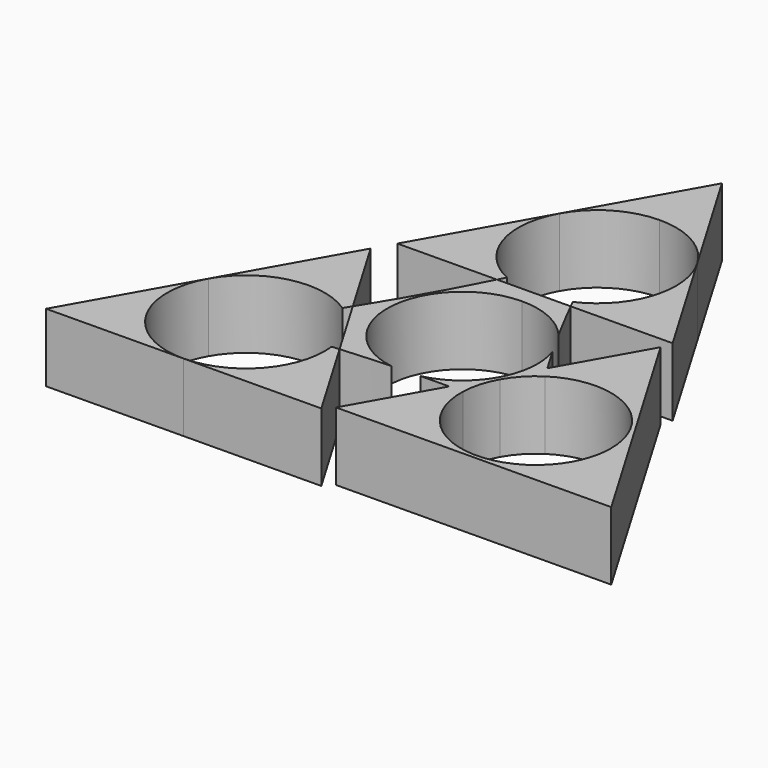
from build123d import *

# Parameters (mm, degrees)
F1_DEPTH = 10


with BuildPart() as f1:
    # F0 (on Top) → F1 (new body)
    with BuildSketch(Plane.XY):
        with BuildLine():
            ThreePointArc((-9.4724629741, -5.5921771434), (-9.5791989557, 5.4073050003), (-0.1067359816, 10.9994821437))
            Line((-0.1067359816, 10.9994821437), (-0.1305380532, 13.4523612782))
            Line((-0.1305380315, 13.4523612785), (-5.6676372798, 13.3986307741))
            ThreePointArc((-5.6676372798, 13.3986307741), (-9.8619346797, 5.5669048062), (-14.3998991761, -2.070826568))
            Line((-14.3998991761, -2.070826568), (-11.5848176191, -6.8392298452))
            Line((-11.5848175812, -6.8392299094), (-9.4724629741, -5.5921771434))
        make_face()
        with BuildLine():
            Line((-0.1305380532, 13.4523612782), (-0.1067359816, 10.9994821437))
            ThreePointArc((-0.1067359816, 10.9994821437), (4.5895542781, 9.9967990641), (8.4111545556, 7.0888982954))
            ThreePointArc((8.4111545556, 7.0888982954), (6.7054289822, 10.2806322034), (5.0577336181, 13.5027068547))
            Line((5.0577336181, 13.5027068547), (-0.1305380315, 13.4523612785))
        make_face()
        with BuildLine():
            ThreePointArc((-1.7230864536, -10.8642060489), (-6.1873786002, -9.0948527233), (-9.4724629741, -5.5921771434))
            Line((-9.4724629741, -5.5921771434), (-11.5848175812, -6.8392299094))
            Line((-11.5848176191, -6.8392298452), (-8.9470811973, -11.3072321903))
            ThreePointArc((-8.9470811973, -11.3072321903), (-5.3370880091, -11.0530388546), (-1.7230864536, -10.8642060489))
        make_face()
    extrude(amount=F1_DEPTH)


with BuildPart() as f1b:
    # F0 (on Top) → F1, piece 2 (new body)
    with BuildSketch(Plane.XY):
        with BuildLine():
            Line((12.5545481824, -0.1363868252), (9.5791989174, -5.4073050681))
            Line((9.5791989557, -5.4073050003), (10.0555510831, -5.6761981773))
            ThreePointArc((10.0555510831, -5.6761981773), (11.606819874, -3.563374371), (13.6139198008, -1.8775484067))
            ThreePointArc((13.6139198008, -1.8775484067), (13.0820160477, -1.0083170753), (12.5545481824, -0.1363868252))
        make_face()
        with BuildLine():
            Line((6.6038497291, -10.6782231755), (9.5791989174, -5.4073050681))
            ThreePointArc((9.5791989174, -5.4073050681), (6.5679269383, -8.8239637201), (2.4308083201, -10.7280553182))
            ThreePointArc((2.4308083201, -10.7280553182), (4.517199042, -10.692254253), (6.6038497291, -10.6782231755))
        make_face()
        with BuildLine():
            Line((10.0555510831, -5.6761981773), (9.5791989557, -5.4073050003))
            Line((9.5791989174, -5.4073050681), (6.6038497291, -10.6782231755))
            ThreePointArc((6.6038497291, -10.6782231755), (7.6229098775, -10.6792833185), (8.6419513958, -10.6855358516))
            ThreePointArc((8.6419513958, -10.6855358516), (9.0481954867, -8.0960523053), (10.0555510831, -5.6761981773))
        make_face()
        with BuildLine():
            ThreePointArc((11, 0), (10.6388718408, -2.7954258985), (9.5791989174, -5.4073050681))
            Line((9.5791989174, -5.4073050681), (12.5545481824, -0.1363868252))
            ThreePointArc((12.5545481824, -0.1363868252), (11.4883643789, 1.6573690273), (10.4409534845, 3.4621511137))
            ThreePointArc((10.4409534845, 3.4621511137), (10.8593390298, 1.7534981708), (11, 0))
        make_face()
        with BuildLine():
            ThreePointArc((8.6419513958, -10.6855358516), (7.6229098775, -10.6792833185), (6.6038497291, -10.6782231755))
            Line((6.6038497291, -10.6782231755), (-0.2522646812, -22.8240303744))
            Line((-0.2522646812, -22.8240303744), (39.7458522051, -22.4358995322))
            Line((39.7458522051, -22.4358995322), (19.4106625927, 12.0094203738))
            Line((19.4106625927, 12.0094203738), (12.5545481824, -0.1363868252))
            ThreePointArc((12.5545481824, -0.1363868252), (13.0820160477, -1.0083170753), (13.6139198008, -1.8775484067))
            ThreePointArc((13.6139198008, -1.8775484067), (24.8678594101, -1.4080411055), (30.6347500389, -11.0835031776))
            ThreePointArc((30.6347500389, -11.0835031776), (30.2736218896, -13.8789290385), (29.2139489946, -16.4908081779))
            ThreePointArc((29.2139489946, -16.4908081779), (16.6472991665, -21.6700577298), (8.6419513958, -10.6855358516))
        make_face()
    extrude(amount=F1_DEPTH)


with BuildPart() as f1c:
    # F0 (on Top) → F1, piece 3 (new body)
    with BuildSketch(Plane.XY):
        with BuildLine():
            ThreePointArc((-5.6676372798, 13.3986307741), (-5.3835781261, 13.9607653638), (-5.1012906228, 14.5237917089))
            ThreePointArc((-5.1012906228, 14.5237917089), (-11.2345943606, 21.4620176196), (-10.2981329222, 30.6750211202))
            Line((-10.2981329222, 30.6750211202), (-20.1295964964, 13.2582958572))
            Line((-20.1295964964, 13.2582958572), (-5.6676372798, 13.3986307741))
        make_face()
    extrude(amount=F1_DEPTH)


with BuildPart() as f1d:
    # F0 (on Top) → F1, piece 4 (new body)
    with BuildSketch(Plane.XY):
        with BuildLine():
            ThreePointArc((11.3044236075, 24.9988230539), (9.473956651, 18.7600560024), (4.5628983325, 14.4992661939))
            ThreePointArc((4.5628983325, 14.4992661939), (4.8096229597, 14.0006424117), (5.0577336181, 13.5027068547))
            Line((5.0577336181, 13.5027068547), (19.8685203899, 13.6464266993))
            Line((19.8685203899, 13.6464266993), (9.7009257177, 30.8690864252))
            ThreePointArc((9.7009257177, 30.8690864252), (10.8963380075, 28.0414862595), (11.3044236075, 24.9988230539))
        make_face()
    extrude(amount=F1_DEPTH)


with BuildPart() as f1e:
    # F0 (on Top) → F1, piece 5 (new body)
    with BuildSketch(Plane.XY):
        with BuildLine():
            ThreePointArc((-8.9470811973, -11.3072321903), (-9.501595119, -11.3520989755), (-10.0559820928, -11.3985080385))
            ThreePointArc((-10.0559820928, -11.3985080385), (-10.0000003021, -12.0529385986), (-9.9813195575, -12.7094935078))
            ThreePointArc((-9.9813195575, -12.7094935078), (-13.3238411908, -20.8347491789), (-21.4162808358, -24.2559552797))
            Line((-21.4162808358, -24.2559552797), (-1.417222775, -24.0618898624))
            Line((-1.417222775, -24.0618898624), (-8.9470811973, -11.3072321903))
        make_face()
    extrude(amount=F1_DEPTH)


with BuildPart() as f1f:
    # F0 (on Top) → F1, piece 6 (new body)
    with BuildSketch(Plane.XY):
        with BuildLine():
            ThreePointArc((-31.5838762413, -7.0332957148), (-24.1799561682, -1.471069011), (-15.0705785167, -3.1370933673))
            ThreePointArc((-15.0705785167, -3.1370933673), (-14.7343993878, -2.6044879851), (-14.3998991761, -2.070826568))
            Line((-14.3998991761, -2.070826568), (-21.7524123874, 10.3834300436))
            Line((-21.7524123874, 10.3834300436), (-31.5838762413, -7.0332957148))
        make_face()
    extrude(amount=F1_DEPTH)


with BuildPart() as f1g:
    # F0 (on Top) → F1, piece 7 (new body)
    with BuildSketch(Plane.XY):
        with BuildLine():
            ThreePointArc((-10.2981329222, 30.6750211202), (-6.1128454296, 34.9423303815), (-0.3546254994, 36.5452848296))
            Line((-0.3546254994, 36.5452848296), (-0.4666692225, 48.0917466053))
            Line((-0.4666692225, 48.0917466053), (-10.2981329222, 30.6750211202))
        make_face()
        with BuildLine():
            Line((-0.4666692225, 48.0917466053), (-0.3546254994, 36.5452848296))
            ThreePointArc((-0.3546254994, 36.5452848296), (5.4336165158, 35.0543740722), (9.7009257177, 30.8690864252))
            Line((9.7009257177, 30.8690864252), (-0.4666692225, 48.0917466053))
        make_face()
    extrude(amount=F1_DEPTH)


with BuildPart() as f1h:
    # F0 (on Top) → F1, piece 8 (new body)
    with BuildSketch(Plane.XY):
        with BuildLine():
            ThreePointArc((-21.4162808358, -24.2559552797), (-27.204522952, -22.7650446849), (-31.4718323013, -18.5797571062))
            Line((-31.4718323013, -18.5797571062), (-41.4153396613, -24.4500207045))
            Line((-41.4153396613, -24.4500207045), (-21.4162808358, -24.2559552797))
        make_face()
        with BuildLine():
            Line((-41.4153396613, -24.4500207045), (-31.4718323013, -18.5797571062))
            ThreePointArc((-31.4718323013, -18.5797571062), (-33.0747867148, -12.8215374515), (-31.5838762413, -7.0332957148))
            Line((-31.5838762413, -7.0332957148), (-41.4153396613, -24.4500207045))
        make_face()
    extrude(amount=F1_DEPTH)


solid = Compound([f1.part, f1b.part, f1c.part, f1d.part, f1e.part, f1f.part, f1g.part, f1h.part])
